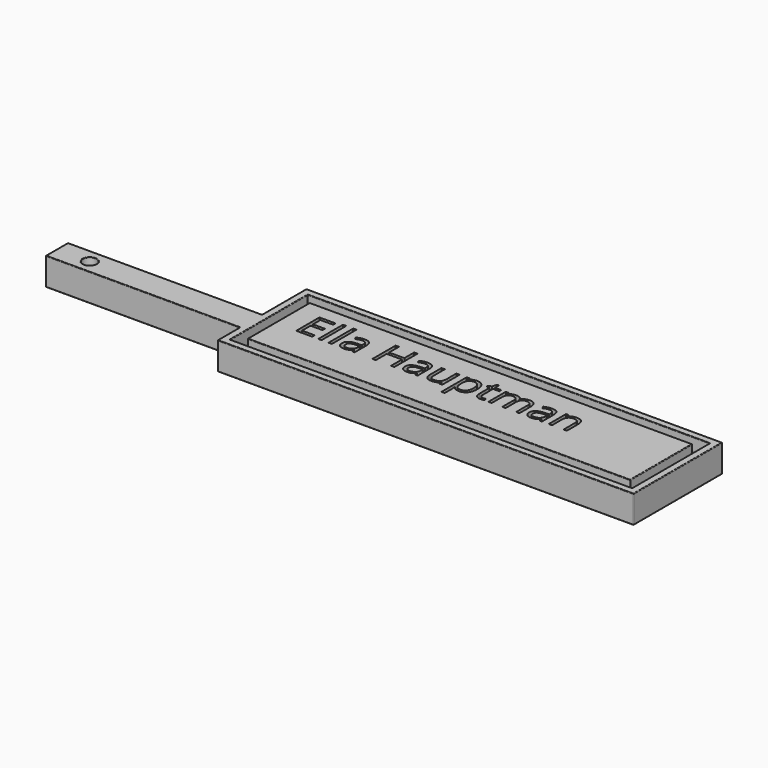
from build123d import *

# Parameters (mm, degrees)
F0_W         = 177.8
F0_H         = 25.4
F1_DEPTH     = 25.4
F2_R         = 6.35
F3_DEPTH     = 25.4
F5_DEPTH     = 12.7
F6_R         = 0.508
F7_TEXT_SIZE = 37.157420741
F8_DEPTH     = 12.7


# Not quite as in the source:
# - Text() gives the source's letters only with a copy of the font that has no kerning and outlines rounded to 1/6400 em; it was checked with that copy


with BuildPart() as f1:
    # F0 (on Top) → F1 (new body)
    with BuildSketch(Plane.XY):
        Polygon((0, 25.4), (0, 0), (381, 0), (381, 101.6), (0, 101.6), (0, 50.8), align=None)
        with Locations((-88.9, 38.1)):
            Rectangle(F0_W, F0_H)
    extrude(amount=F1_DEPTH)

    # F2 (on face) → F3 (cut)
    with BuildSketch(Plane.XY.offset(25.4)):
        with Locations((-147.7334797382, 38.1)):
            Circle(F2_R)
    extrude(amount=-F3_DEPTH, mode=Mode.SUBTRACT)

    # F4 (on face) → F5 (cut)
    with BuildSketch(Plane.XY.offset(25.4)):
        Polygon((374.65, 6.35), (374.65, 95.25), (6.35, 95.25), (6.35, 44.45), (6.35, 31.75), (6.35, 6.35), align=None)
        Polygon((365.76, 86.36), (365.76, 15.24), (15.24, 15.24), (15.24, 31.75), (15.24, 44.45), (15.24, 86.36), align=None, mode=Mode.SUBTRACT)
    extrude(amount=-F5_DEPTH, mode=Mode.SUBTRACT)

    # F6
    f6_edges = [f1.edges().sort_by_distance(p)[0] for p in [
        (0, 0, 12.7),
        (381, 0, 12.7),
        (190.5, 0, 0),
        (190.5, 0, 25.4),
        (381, 101.6, 12.7),
        (0, 101.6, 12.7),
        (190.5, 101.6, 0),
        (190.5, 101.6, 25.4),
        (0, 50.8, 12.7),
        (0, 76.2, 0),
        (0, 76.2, 25.4),
        (381, 50.8, 0),
        (381, 50.8, 25.4),
        (-177.8, 50.8, 12.7),
        (-88.9, 50.8, 0),
        (-88.9, 50.8, 25.4),
        (-177.8, 25.4, 12.7),
        (0, 25.4, 12.7),
        (-88.9, 25.4, 0),
        (-88.9, 25.4, 25.4),
        (-177.8, 38.1, 0),
        (-177.8, 38.1, 25.4),
        (-141.38348, 38.1, 12.7),
        (-154.08348, 38.1, 25.4),
        (-154.08348, 38.1, 0),
        (374.65, 95.25, 19.05),
        (6.35, 95.25, 19.05),
        (190.5, 95.25, 25.4),
        (190.5, 95.25, 12.7),
        (190.5, 6.35, 12.7),
        (374.65, 50.8, 12.7),
        (6.35, 50.8, 12.7),
        (190.5, 86.36, 12.7),
        (365.76, 50.8, 12.7),
        (190.5, 15.24, 12.7),
        (15.24, 50.8, 12.7),
        (374.65, 6.35, 19.05),
        (374.65, 50.8, 25.4),
        (6.35, 6.35, 19.05),
        (6.35, 50.8, 25.4),
        (190.5, 6.35, 25.4),
        (365.76, 86.36, 19.05),
        (365.76, 15.24, 19.05),
        (365.76, 50.8, 25.4),
        (15.24, 15.24, 19.05),
        (15.24, 86.36, 19.05),
        (15.24, 50.8, 25.4),
        (190.5, 86.36, 25.4),
        (190.5, 15.24, 25.4),
        (0, 12.7, 25.4),
        (0, 12.7, 0),
    ]]
    fillet(f6_edges, radius=F6_R)

    # F7 (on face) → F8 (cut)
    with BuildSketch(Plane.XY.offset(25.4)):
        with Locations((31.242, 46.3986570664)):
            Text('Ella Hauptman', F7_TEXT_SIZE, font='Open Sans', text_align=(TextAlign.LEFT, TextAlign.BOTTOM))
    extrude(amount=-F8_DEPTH, mode=Mode.SUBTRACT)


solid = f1.part
